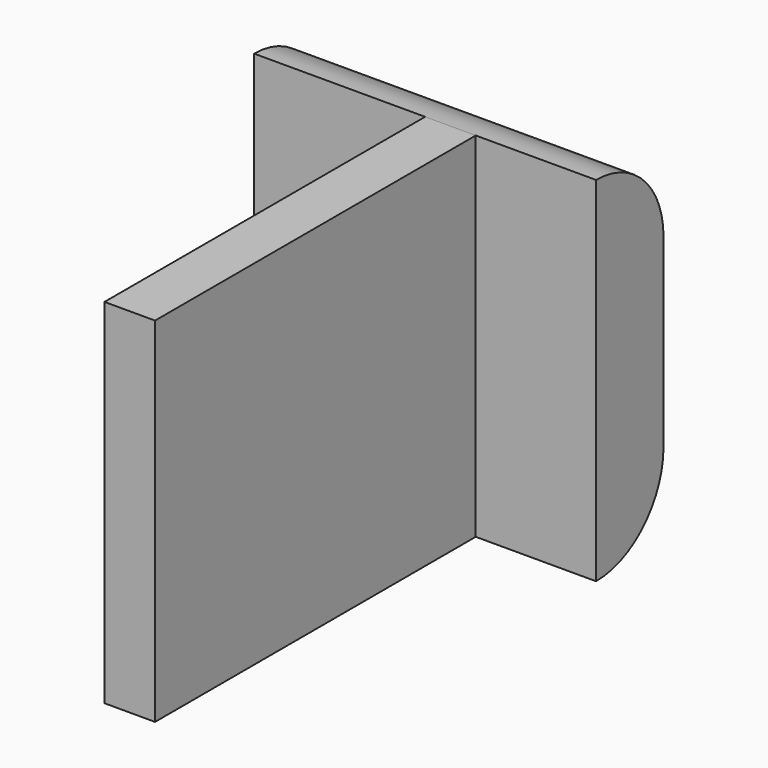
from build123d import *

# Parameters (mm, degrees)
F1_E1_RIGHT_W = 20.9673028439
F1_E1_RIGHT_H = 23.7872338621
F2_DEPTH      = 3
F0_W          = 10.1448968053
F0_H          = 20.9673028439
F3_DEPTH      = 5
F4_R          = 5
F5_R          = 5


with BuildPart() as f2:
    # F1_E1_right (on explicit) → F2 (new body)
    with BuildSketch(Plane(origin=(-10.1448968053, 0, 16.1632616073), x_dir=(0, 0, 1), z_dir=(1, 0, 0))):
        with Locations((10.483651422, 11.893616931)):
            Rectangle(F1_E1_RIGHT_W, F1_E1_RIGHT_H)
    extrude(amount=F2_DEPTH)

    # F0 (on Front) → F3 (join)
    with BuildSketch(Plane.XZ):
        with Locations((-5.0724484026, 26.6469130293)):
            Rectangle(F0_W, F0_H)
        with Locations((-15.2173452079, 26.6469130293)):
            Rectangle(F0_W, F0_H)
    extrude(amount=-F3_DEPTH)

    # F4
    f4_edges = [f2.edges().sort_by_distance(p)[0] for p in [
        (-10.144897, 5, 37.130564),
    ]]
    fillet(f4_edges, radius=F4_R)

    # F5
    f5_edges = [f2.edges().sort_by_distance(p)[0] for p in [
        (-10.144897, 5, 16.163262),
    ]]
    fillet(f5_edges, radius=F5_R)


solid = f2.part
